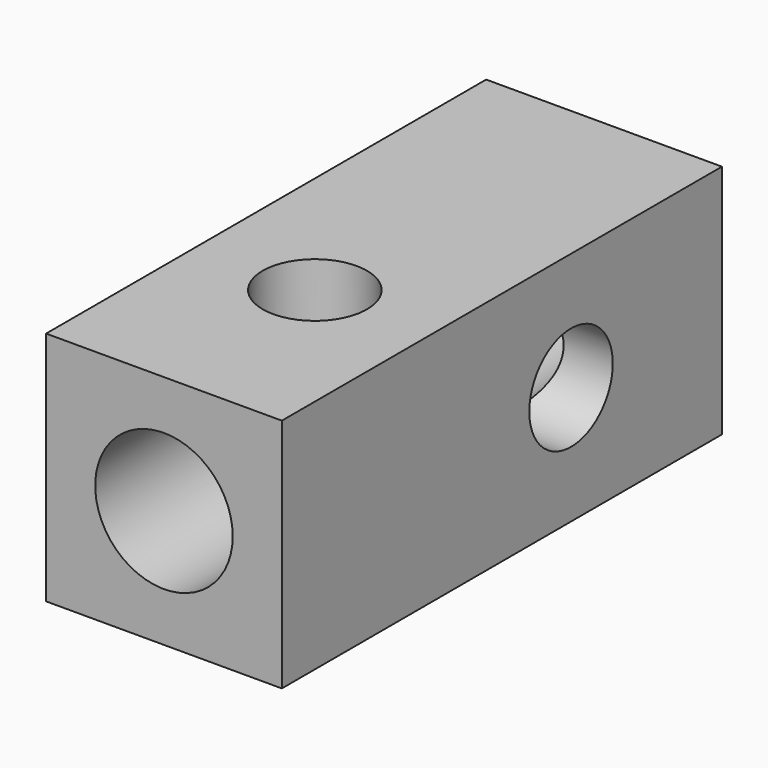
from build123d import *

# Parameters (mm, degrees)
F0_W     = 19.05
F0_H     = 19.05
F0_R     = 5.55625
F1_DEPTH = 44.45
F3_D     = 8.4328
F5_D     = 8.4328


# Not quite as in the source:
# - a feature names something its author has since deleted; it is built from what else it names


with BuildPart() as f1:
    # F0 (on Front) → F1 (new body)
    with BuildSketch(Plane.XZ):
        with Locations((9.525, 9.525)):
            Rectangle(F0_W, F0_H)
        with Locations((9.525, 9.525)):
            Circle(F0_R, mode=Mode.SUBTRACT)
    extrude(amount=F1_DEPTH)

    # F3 (through all)
    with Locations(Plane.XY.offset(19.05)):
        with Locations((9.525, -29.21)):
            Hole(F3_D / 2)

    # F5 (through all)
    with Locations(Plane.YZ.offset(19.05)):
        with Locations((-15.24, 9.525)):
            Hole(F5_D / 2)


solid = f1.part
